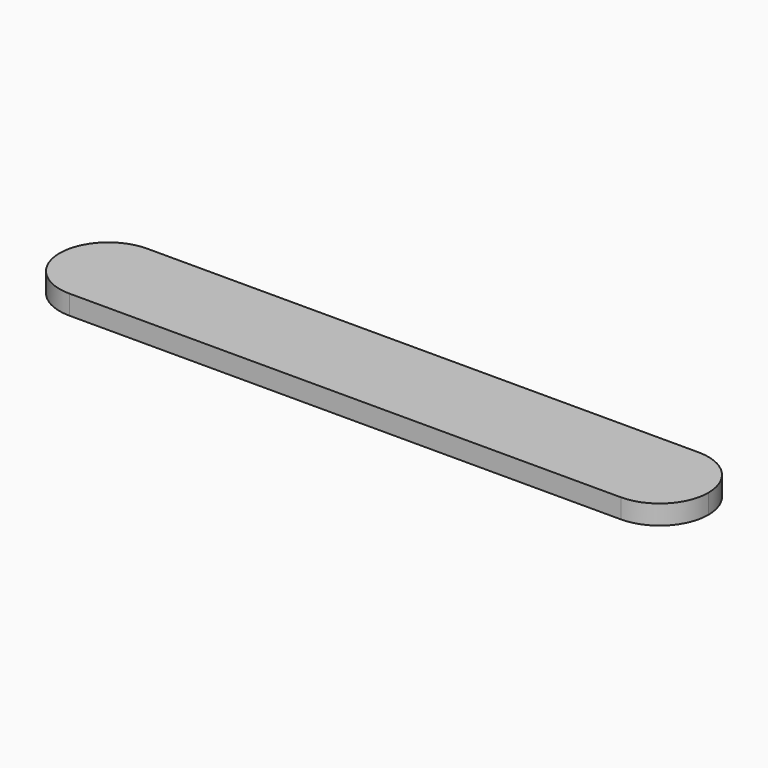
from build123d import *

# Parameters (mm, degrees)
F0_W     = 50.8
F0_H     = 7.62
F1_DEPTH = 1.524
F2_R     = 3.80999


# Not quite as in the source:
# - a fillet or chamfer is up to 0.001 mm smaller than in the source, because OpenCascade refuses the exact size


with BuildPart() as f1:
    # F0 (on Top) → F1 (new body)
    with BuildSketch(Plane.XY):
        Rectangle(F0_W, F0_H)
    extrude(amount=F1_DEPTH)

    # F2 (radius 3.81 in the source; OpenCascade refuses exactly that, so slightly less here)
    f2_edges = [f1.edges().sort_by_distance(p)[0] for p in [
        (25.4, 3.81, 0.762),
        (25.4, -3.81, 0.762),
        (-25.4, -3.81, 0.762),
        (-25.4, 3.81, 0.762),
    ]]
    fillet(f2_edges, radius=F2_R)


solid = f1.part
